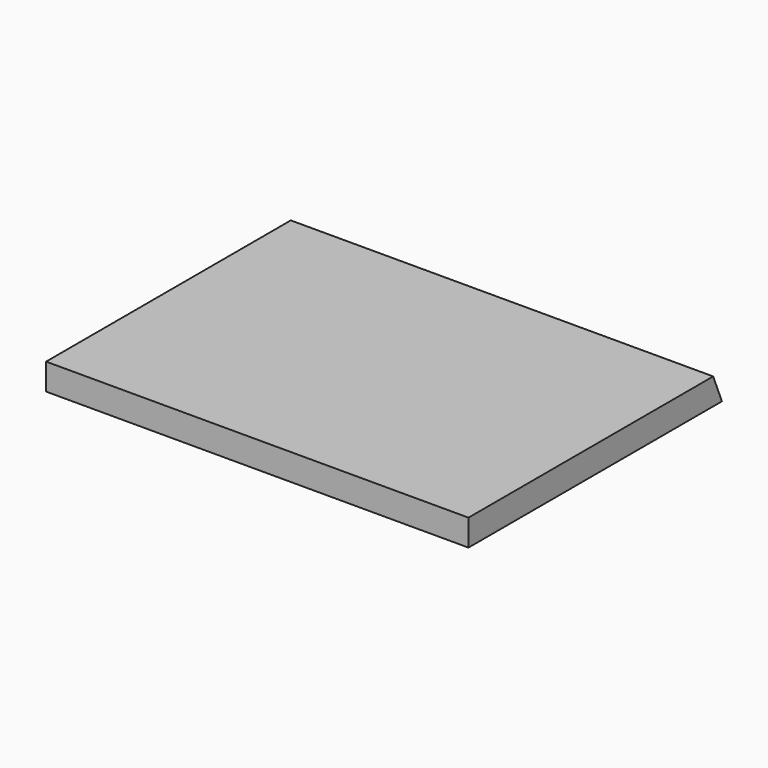
from build123d import *

# Parameters (mm, degrees)
F0_W     = 304.8
F0_H     = 228.6
F1_DEPTH = 19.05
F2_SIZE2 = 7.890758
F2_SIZE  = 19.04999


# Not quite as in the source:
# - a fillet or chamfer is up to 0.001 mm smaller than in the source, because OpenCascade refuses the exact size


with BuildPart() as f1:
    # F0 (on Top) → F1 (new body)
    with BuildSketch(Plane.XY):
        Rectangle(F0_W, F0_H)
    extrude(amount=F1_DEPTH)

    # F2 (size 19.05 and 7.8907683632 in the source; OpenCascade refuses exactly that, so slightly less here)
    f2_edges = [f1.edges().sort_by_distance(p)[0] for p in [
        (0, 114.3, 19.05),
    ]]
    f2_side = f1.faces().sort_by_distance((0, 114.3, 9.525))[0]
    chamfer(f2_edges, length=F2_SIZE, length2=F2_SIZE2, reference=f2_side)


solid = f1.part
